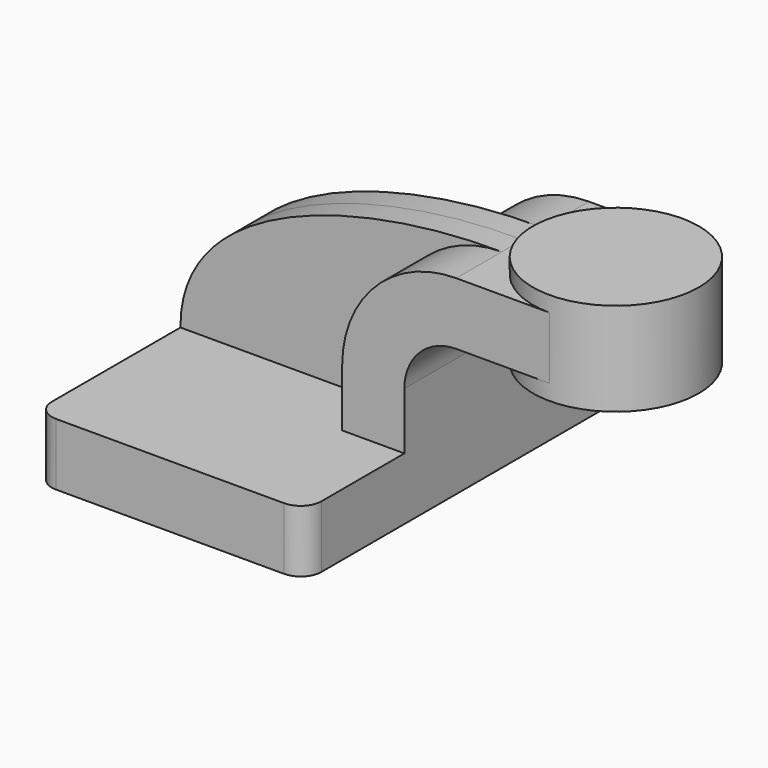
from build123d import *

# Parameters (mm, degrees)
F1_DEPTH = 63.5
F0_W     = 25.4
F0_H     = 19.05
F2_DEPTH = 25.4
F3_DEPTH = 7.9375
F5_R     = 6.35


# Not quite as in the source:
# - a feature names something its author has since deleted; it is built from what else it names


with BuildPart() as f1:
    # F0 (on Front) → F1 (new body, symmetric)
    with BuildSketch(Plane.XZ):
        Polygon((-41.275, 9.525), (-41.275, -9.525), (41.275, -9.525), (41.275, 9.525), (22.225, 9.525), align=None)
    extrude(amount=F1_DEPTH, both=True)

    # F0 (on Front) → F2 (join, symmetric)
    with BuildSketch(Plane.XZ):
        with BuildLine():
            Line((22.225, 9.525), (41.275, 9.525))
            Line((41.275, 9.525), (41.275, 27.0002))
            ThreePointArc((41.275, 27.0002), (45.9246798487, 38.2255201513), (57.15, 42.8752))
            Line((57.15, 42.8752), (60.325, 42.8752))
            Line((60.325, 42.8752), (60.325, 61.9252))
            Line((60.325, 61.9252), (57.15, 61.9252))
            ThreePointArc((57.15, 61.9252), (32.4542956671, 51.6959043329), (22.225, 27.0002))
            Line((22.225, 27.0002), (22.225, 9.525))
        make_face()
        with Locations((73.025, 52.4002)):
            Rectangle(F0_W, F0_H)
    extrude(amount=F2_DEPTH, both=True)

    # F0 (on Front) → F3 (join, symmetric)
    with BuildSketch(Plane.XZ):
        with BuildLine():
            add(Edge.make_bspline(
                [(-41.275, 9.525), (-41.515853256, 47.6718097925), (16.0763282329, 62.4862834811), (57.15, 61.9252)],
                knots=[0, 0, 0, 0, 111.5045361635, 111.5045361635, 111.5045361635, 111.5045361635], degree=3))
            Line((-41.275, 9.525), (22.225, 9.525))
            Line((22.225, 9.525), (22.225, 27.0002))
            ThreePointArc((22.225, 27.0002), (32.4542956671, 51.6959043329), (57.15, 61.9252))
        make_face()
    extrude(amount=F3_DEPTH, both=True)

    # F0 (on Front) → F4 (revolve)
    with BuildSketch(Plane.XZ):
        Polygon((85.725, 66.675), (85.725, 61.9252), (85.725, 42.8752), (85.725, 38.1), (111.125, 38.1), (111.125, 66.675), align=None)
    revolve(axis=Axis((85.725, 0, 52.3875), (0, 0, 1)))

    # F5
    f5_edges = [f1.edges().sort_by_distance(p)[0] for p in [
        (-41.275, -63.5, 0),
        (41.275, -63.5, 0),
        (41.275, 63.5, 0),
        (-41.275, 63.5, 0),
    ]]
    fillet(f5_edges, radius=F5_R)


solid = f1.part
